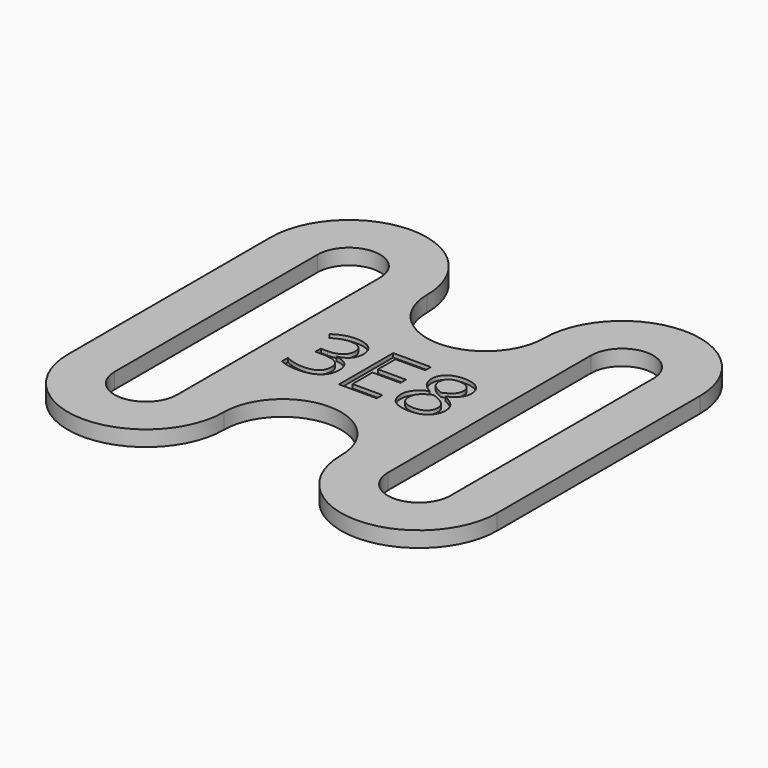
from build123d import *

# Parameters (mm, degrees)
F1_DEPTH     = 2
F2_TEXT_SIZE = 12.1527777778
F3_DEPTH     = 0.5


# Not quite as in the source:
# - Text() gives the source's letters only with a copy of the font that has no kerning and outlines rounded to 1/6400 em; it was checked with that copy


with BuildPart() as f1:
    # F0 (on Top) → F1 (new body)
    with BuildSketch(Plane.XY):
        with BuildLine():
            ThreePointArc((7.5, 16.25), (0, 8.75), (-7.5, 16.25))
            ThreePointArc((-7.5, 16.25), (-17.5, 26.25), (-27.5, 16.25))
            Line((-27.5, 16.25), (-27.5, -16.25))
            ThreePointArc((-27.5, -16.25), (-17.5, -26.25), (-7.5, -16.25))
            ThreePointArc((-7.5, -16.25), (0, -8.75), (7.5, -16.25))
            ThreePointArc((7.5, -16.25), (17.5, -26.25), (27.5, -16.25))
            Line((27.5, -16.25), (27.5, 16.25))
            ThreePointArc((27.5, 16.25), (17.5, 26.25), (7.5, 16.25))
        make_face()
        with BuildLine():
            ThreePointArc((-21.5, 16.25), (-17.5, 20.25), (-13.5, 16.25))
            Line((-13.5, 16.25), (-13.5, -16.25))
            ThreePointArc((-13.5, -16.25), (-17.5, -20.25), (-21.5, -16.25))
            Line((-21.5, -16.25), (-21.5, 16.25))
        make_face(mode=Mode.SUBTRACT)
        with BuildLine():
            Line((13.5, -16.25), (13.5, 16.25))
            ThreePointArc((13.5, 16.25), (17.5, 20.25), (21.5, 16.25))
            Line((21.5, 16.25), (21.5, -16.25))
            ThreePointArc((21.5, -16.25), (17.5, -20.25), (13.5, -16.25))
        make_face(mode=Mode.SUBTRACT)
    extrude(amount=F1_DEPTH)

    # F2 (on face) → F3 (cut)
    with BuildSketch(Plane.XY.offset(2)):
        with Locations((-10.406765408, -4.375)):
            Text('3E8', F2_TEXT_SIZE, font='Open Sans', text_align=(TextAlign.LEFT, TextAlign.BOTTOM))
    extrude(amount=-F3_DEPTH, mode=Mode.SUBTRACT)


solid = f1.part
